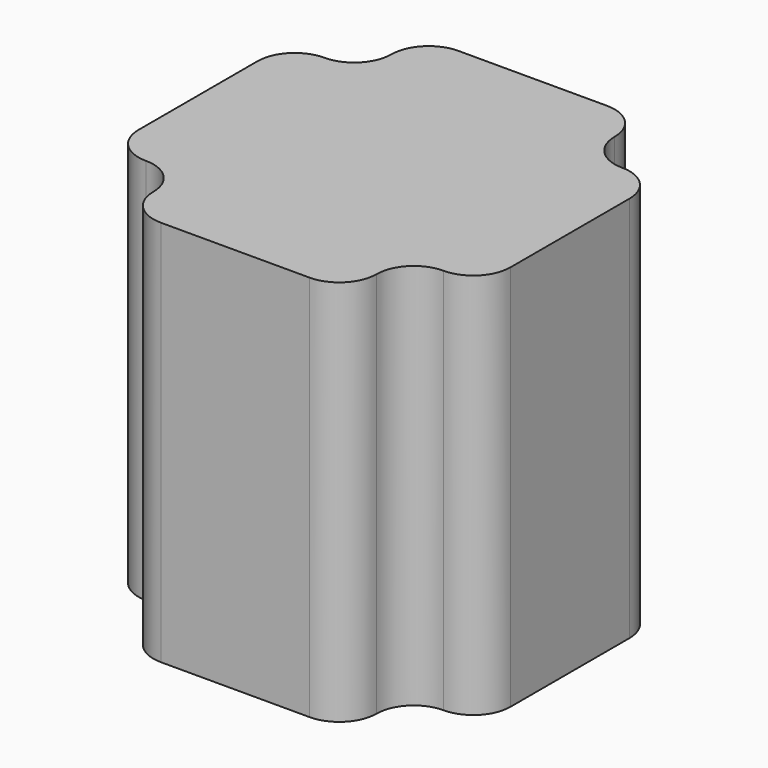
from build123d import *

# Parameters (mm, degrees)
F1_DEPTH = 52
F2_R     = 5
F3_R     = 4.99999


# Not quite as in the source:
# - a fillet or chamfer is up to 0.001 mm smaller than in the source, because OpenCascade refuses the exact size


with BuildPart() as f1:
    # F0 (on Top) → F1 (new body)
    with BuildSketch(Plane.XY):
        Polygon((15, 25), (-15, 25), (-15, 15), (-25, 15), (-25, -15), (-15, -15), (-15, -25), (15, -25), (15, -15), (25, -15), (25, 15), (15, 15), align=None)
    extrude(amount=F1_DEPTH)

    # F2
    f2_edges = [f1.edges().sort_by_distance(p)[0] for p in [
        (-15, -15, 26),
        (15, -15, 26),
        (15, 15, 26),
        (-15, 15, 26),
    ]]
    fillet(f2_edges, radius=F2_R)

    # F3 (radius 5 in the source; OpenCascade refuses exactly that, so slightly less here)
    f3_edges = [f1.edges().sort_by_distance(p)[0] for p in [
        (25, 15, 26),
        (-15, 25, 26),
        (-25, 15, 26),
        (25, -15, 26),
        (15, -25, 26),
        (-15, -25, 26),
        (-25, -15, 26),
        (15, 25, 26),
    ]]
    fillet(f3_edges, radius=F3_R)


solid = f1.part
